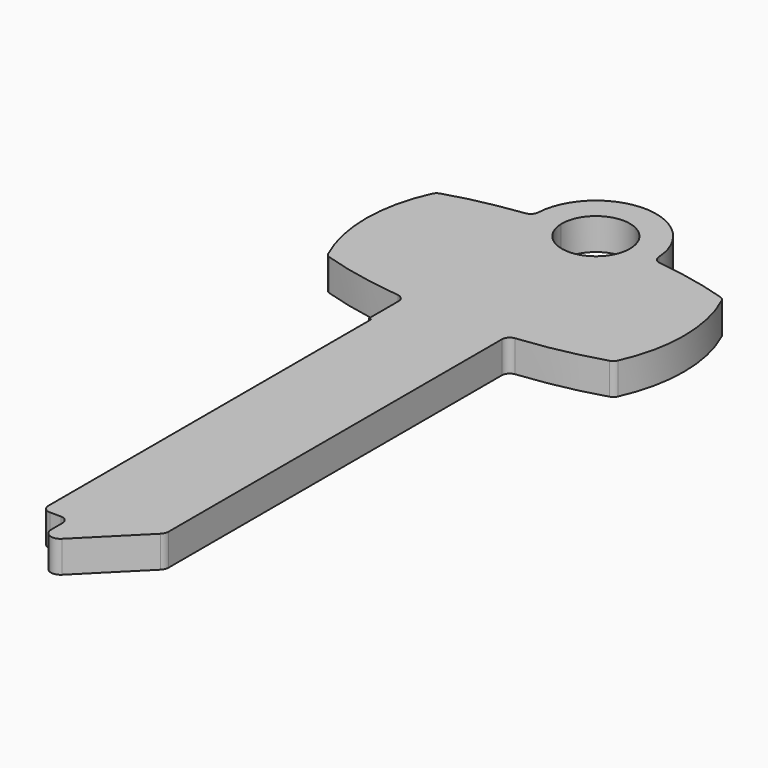
from build123d import *

# Parameters (mm, degrees)
F1_DEPTH = 2.54
F3_DEPTH = 2.54
F4_R     = 0.635


with BuildPart() as f1:
    # F0 (on Top) → F1 (new body)
    with BuildSketch(Plane.XY):
        with BuildLine():
            ThreePointArc((2.7292355161, -0.0830887952), (0, -2.7305), (-2.7292355161, -0.0830887952))
            add(Edge.make_bspline(
                [(-2.7292355161, -0.0830887952), (-3.7940557667, -0.1483067369), (-4.8315057716, -0.2637606285)],
                knots=[1.7238043068, 1.7238043068, 1.7238043068, 1.8439930848, 1.8439930848, 1.8439930848], degree=2, weights=[1, 0.9981948755, 1]))
            add(Edge.make_bspline(
                [(-4.8315057716, -0.2637606285), (-8.5391367, -0.6763688673), (-11.4920446345, -1.6577838797)],
                knots=[1.8439930848, 1.8439930848, 1.8439930848, 2.2675908503, 2.2675908503, 2.2675908503], degree=2, weights=[1, 0.9776543376, 1]))
            ThreePointArc((-11.4920446345, -1.6577838797), (-12.7508, -7.112), (-11.4920446345, -12.5662161203))
            add(Edge.make_bspline(
                [(-11.4920446345, -12.5662161203), (0, -16.3856596579), (11.4920446345, -12.5662161203)],
                knots=[4.0155944569, 4.0155944569, 4.0155944569, 5.4091835039, 5.4091835039, 5.4091835039], degree=2, weights=[1, 0.766903279, 1]))
            ThreePointArc((11.4920446345, -12.5662161203), (12.7508, -7.112), (11.4920446345, -1.6577838797))
            add(Edge.make_bspline(
                [(11.4920446345, -1.6577838797), (8.5391367, -0.6763688673), (4.8315057716, -0.2637606285)],
                knots=[0.8740018033, 0.8740018033, 0.8740018033, 1.2975995688, 1.2975995688, 1.2975995688], degree=2, weights=[1, 0.9776543376, 1]))
            add(Edge.make_bspline(
                [(4.8315057716, -0.2637606285), (3.7940557667, -0.1483067369), (2.7292355161, -0.0830887952)],
                knots=[1.2975995688, 1.2975995688, 1.2975995688, 1.4177883468, 1.4177883468, 1.4177883468], degree=2, weights=[1, 0.9981948755, 1]))
        make_face()
        with BuildLine():
            ThreePointArc((-2.7292355161, -0.0830887952), (-0.0415492082, 2.7301838607), (2.7305, 0))
            ThreePointArc((2.7305, 0), (2.7301838607, -0.0415492082), (2.7292355161, -0.0830887952))
            add(Edge.make_bspline(
                [(4.8315057716, -0.2637606285), (3.7940557667, -0.1483067369), (2.7292355161, -0.0830887952)],
                knots=[1.2975995688, 1.2975995688, 1.2975995688, 1.4177883468, 1.4177883468, 1.4177883468], degree=2, weights=[1, 0.9981948755, 1]))
            ThreePointArc((4.8315057716, -0.2637606285), (0, 4.8387), (-4.8315057716, -0.2637606285))
            add(Edge.make_bspline(
                [(-2.7292355161, -0.0830887952), (-3.7940557667, -0.1483067369), (-4.8315057716, -0.2637606285)],
                knots=[1.7238043068, 1.7238043068, 1.7238043068, 1.8439930848, 1.8439930848, 1.8439930848], degree=2, weights=[1, 0.9981948755, 1]))
        make_face()
    extrude(amount=F1_DEPTH)

    # F2 (on Top) → F3 (join, through all)
    with BuildSketch(Plane.XY):
        with BuildLine():
            add(Edge.make_bspline(
                [(-4.1402, -14.0312996195), (0, -14.4220670272), (4.1402, -14.0312996195)],
                knots=[4.4790722282, 4.4790722282, 4.4790722282, 4.9457057325, 4.9457057325, 4.9457057325], degree=2, weights=[1, 0.9729048959, 1]))
            Line((-4.1402, -14.0312996195), (-4.1402, -17.5872996195))
            Line((-4.1402, -17.5872996195), (-3.937, -17.5872996195))
            Line((-3.937, -17.5872996195), (-3.937, -50.6072996195))
            Line((-3.937, -50.6072996195), (-1.778, -50.6072996195))
            Line((-1.778, -50.6072996195), (-1.778, -52.3998688849))
            ThreePointArc((-1.778, -52.3998688849), (-1.3076047755, -53.1038650887), (-0.4771846327, -52.9386842522))
            Line((-0.4771846327, -52.9386842522), (3.9170153673, -48.5444842522))
            ThreePointArc((3.9170153673, -48.5444842522), (4.0821962038, -48.2972736604), (4.1402, -48.0056688849))
            Line((4.1402, -48.0056688849), (4.1402, -14.0312996195))
        make_face()
    extrude(amount=F3_DEPTH)

    # F4
    f4_edges = [f1.edges().sort_by_distance(p)[0] for p in [
        (-4.1402, -14.0313, 1.27),
        (4.1402, -14.0313, 1.27),
        (11.492045, -12.566216, 1.27),
        (11.492045, -1.657784, 1.27),
        (-11.492045, -1.657784, 1.27),
        (-11.492045, -12.566216, 1.27),
        (-3.937, -50.6073, 1.27),
        (-1.778, -50.6073, 1.27),
        (4.831506, -0.263761, 1.27),
        (-4.831506, -0.263761, 1.27),
    ]]
    fillet(f4_edges, radius=F4_R)


solid = f1.part
